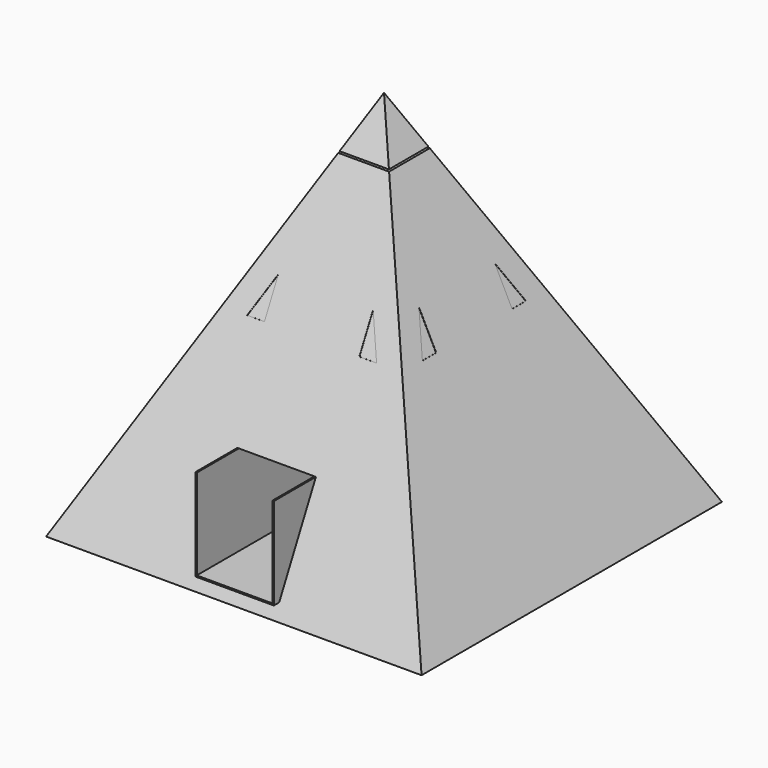
from build123d import *

# Parameters (mm, degrees)
F0_W             = 75.7989510894
F0_H             = 76.0997384787
F1_DEPTH         = 76.2
F2_W             = 94.859868288
F2_H             = 5.5733323097
F3_DEPTH         = 81.28
F5_DEPTH         = 81.28
F7_W             = 38.1
F7_H             = 38.1
F14_W            = 33.9892096817
F14_H            = 0.3007873893
F15_DEPTH        = 254
F15_DEPTH_BACK   = 127
F17_DEPTH        = 0.0508
F17_COPIES_COUNT = 4
F19_W            = 15.9418433905
F19_H            = 18.6489464249
F20_DEPTH        = 38.1
F21_W            = 15.3402625583
F21_H            = 18.348157173
F22_DEPTH        = 101.6


# Not quite as in the source:
# - a pattern or mirror of a feature is missing from the dataset's text; its kind, count and spacing are read off the source's solid


with BuildPart() as f1:
    # F0 (on Front) → F1 (new body)
    with BuildSketch(Plane.XZ):
        with Locations((37.8994755447, -38.0498692393)):
            Rectangle(F0_W, F0_H)
    extrude(amount=F1_DEPTH)

    # F2 (on face) → F3 (cut)
    with BuildSketch(Plane.XZ.offset(76.2)):
        with Locations((-47.429934144, -78.8864046335)):
            Rectangle(F2_W, F2_H)
        Polygon((0, 0), (0, -76.0997384787), (37.8994755447, 0), align=None)
    extrude(amount=-F3_DEPTH, mode=Mode.SUBTRACT)

    # F4 (on face) → F5 (cut)
    with BuildSketch(Plane.XZ.offset(76.2)):
        Polygon((75.7989510894, 0), (37.8994755447, 0), (75.7989510894, -76.0997384787), align=None)
    extrude(amount=-F5_DEPTH, mode=Mode.SUBTRACT)


with BuildPart() as f10:
    # F7 (on Top) → F10 section 0
    with BuildSketch(Plane.XY, mode=Mode.PRIVATE) as f10_s0:
        with Locations((-19.05, 19.05)):
            Rectangle(F7_W, F7_H)
    loft([f10_s0.sketch, Vertex(0, 0, 76.2)])

    # F7 (on Top) → F11 section 0
    with BuildSketch(Plane.XY, mode=Mode.PRIVATE) as f11_s0:
        with Locations((-19.05, -19.05)):
            Rectangle(F7_W, F7_H)
    loft([f11_s0.sketch, Vertex(0, 0, 76.2)])

    # F7 (on Top) → F12 section 0
    with BuildSketch(Plane.XY, mode=Mode.PRIVATE) as f12_s0:
        with Locations((19.05, -19.05)):
            Rectangle(F7_W, F7_H)
    loft([f12_s0.sketch, Vertex(0, 0, 76.2)])

    # F7 (on Top) → F13 section 0
    with BuildSketch(Plane.XY, mode=Mode.PRIVATE) as f13_s0:
        with Locations((19.05, 19.05)):
            Rectangle(F7_W, F7_H)
    loft([f13_s0.sketch, Vertex(0, 0, 76.2)])

    # F14 (on Front) → F15 (cut, two sides)
    with BuildSketch(Plane.XZ) as f15_sk:
        with Locations((0.4511848092, 66.0232938826)):
            Rectangle(F14_W, F14_H)
    extrude(amount=-F15_DEPTH, mode=Mode.SUBTRACT)
    extrude(f15_sk.sketch, amount=F15_DEPTH_BACK, mode=Mode.SUBTRACT)

    # F16 (on face) → F17 (cut)
    with BuildSketch(Plane(origin=(30.48, 0, 15.24), x_dir=(0, 1, 0), z_dir=(0.894427191, 0, 0.4472135955))):
        Polygon((-9.6252635121, 27.2397237785), (-9.6252635121, 35.0865572691), (-13.1344741307, 27.2397237785), align=None)
    f17 = extrude(amount=-F17_DEPTH, mode=Mode.SUBTRACT)

    # F17_copies: F17 ×4 about axis
    f17_copies_axis = Axis((0, 0, 0), (0, 0, 1))
    for i in range(1, F17_COPIES_COUNT):
        add(f17.rotate(f17_copies_axis, i * 360 / F17_COPIES_COUNT), mode=Mode.SUBTRACT)

    # F17_copies1: F17 across plane
    add(f17.mirror(Plane(origin=(0, 0, 0), x_dir=(-0.7071067812, -0.7071067812, 0), z_dir=(-0.7071067812, 0.7071067812, 0))), mode=Mode.SUBTRACT)

    # F17_copies2: F17 across plane
    add(f17.mirror(Plane(origin=(0, 0, 0), x_dir=(0, 0, -1), z_dir=(-1, 0, 0))), mode=Mode.SUBTRACT)

    # F17_copies3: F17 across plane
    add(f17.mirror(Plane(origin=(0, 0, 0), x_dir=(0.7071067812, -0.7071067812, 0), z_dir=(-0.7071067812, -0.7071067812, 0))), mode=Mode.SUBTRACT)

    # F17_copies4: F17 across plane
    add(f17.mirror(Plane.ZX), mode=Mode.SUBTRACT)

    # F19 (on Front) → F20 (join)
    with BuildSketch(Plane.XZ):
        with Locations((0.150394626, 12.0315785753)):
            Rectangle(F19_W, F19_H)
    extrude(amount=F20_DEPTH)

    # F21 (on Front) → F22 (cut)
    with BuildSketch(Plane.XZ):
        with Locations((0.1503948588, 12.1819732012)):
            Rectangle(F21_W, F21_H)
    extrude(amount=F22_DEPTH, mode=Mode.SUBTRACT)


solid = f10.part
